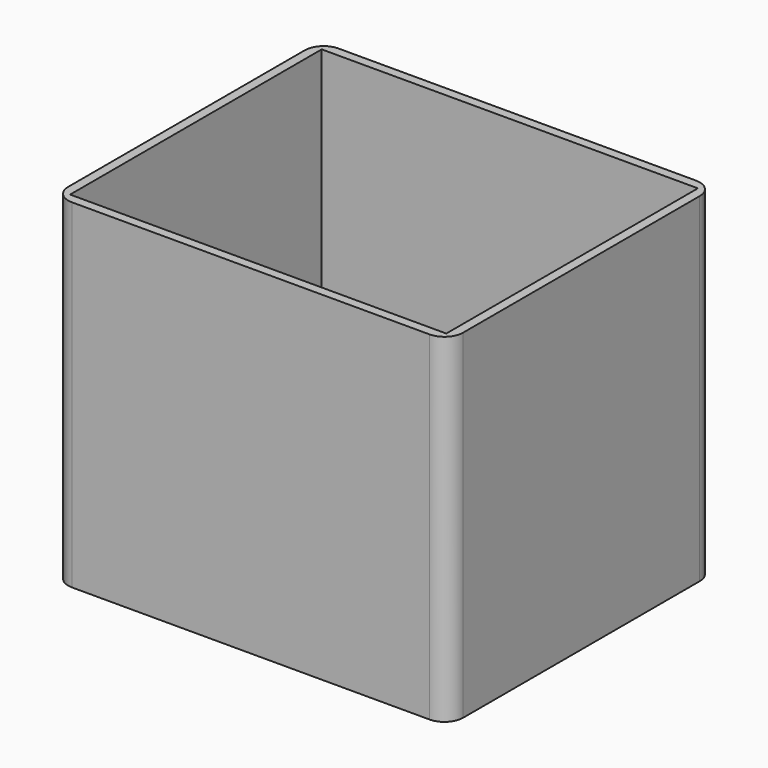
from build123d import *

# Parameters (mm, degrees)
F0_W        = 102.4
F0_H        = 85.6
F1_DEPTH    = 89.75
F2_T        = 2.54
F3_T1_DEPTH = 117.69


# Not quite as in the source:
# - a fillet or chamfer that OpenCascade refuses, or shapes differently, is made with other operations: its cross-section is extruded or revolved along the edge and cut away or added


with BuildPart() as f1:
    # F0 (on Top) → F1 (new body)
    with BuildSketch(Plane.XY):
        with Locations((0.6768562123, 7.1260996301)):
            Rectangle(F0_W, F0_H)
    extrude(amount=F1_DEPTH)

    # F2
    f2_openings = [f1.faces().sort_by_distance(p)[0] for p in [
        (0.676856, 7.1261, 89.75),
    ]]
    offset(amount=F2_T, openings=f2_openings, kind=Kind.INTERSECTION)

    # F3: fillet of radius 5.08 on 4 edges, made by hand

    # F3_s2 → F3_t1 (cut)
    with BuildSketch(Plane.XY.offset(-15.24)):
        with BuildLine():
            ThreePointArc((49.3368562123, 52.4660996301), (52.9289586607, 50.9782020785), (54.4168562123, 47.3860996301))
            Line((54.4168562123, 47.3860996301), (54.4168562123, 52.4660996301))
            Line((54.4168562123, 52.4660996301), (49.3368562123, 52.4660996301))
        make_face()
        with BuildLine():
            ThreePointArc((-47.9831437877, 52.4660996301), (-51.5752462361, 50.9782020785), (-53.0631437877, 47.3860996301))
            Line((-53.0631437877, 47.3860996301), (-53.0631437877, 52.4660996301))
            Line((-53.0631437877, 52.4660996301), (-47.9831437877, 52.4660996301))
        make_face()
        with BuildLine():
            ThreePointArc((-53.0631437877, -33.1339003699), (-51.5752462361, -36.7260028183), (-47.9831437877, -38.2139003699))
            Line((-47.9831437877, -38.2139003699), (-53.0631437877, -38.2139003699))
            Line((-53.0631437877, -38.2139003699), (-53.0631437877, -33.1339003699))
        make_face()
        with BuildLine():
            ThreePointArc((49.3368562123, -38.2139003699), (52.9289586607, -36.7260028183), (54.4168562123, -33.1339003699))
            Line((54.4168562123, -33.1339003699), (54.4168562123, -38.2139003699))
            Line((54.4168562123, -38.2139003699), (49.3368562123, -38.2139003699))
        make_face()
    extrude(amount=F3_T1_DEPTH, mode=Mode.SUBTRACT)


solid = f1.part
